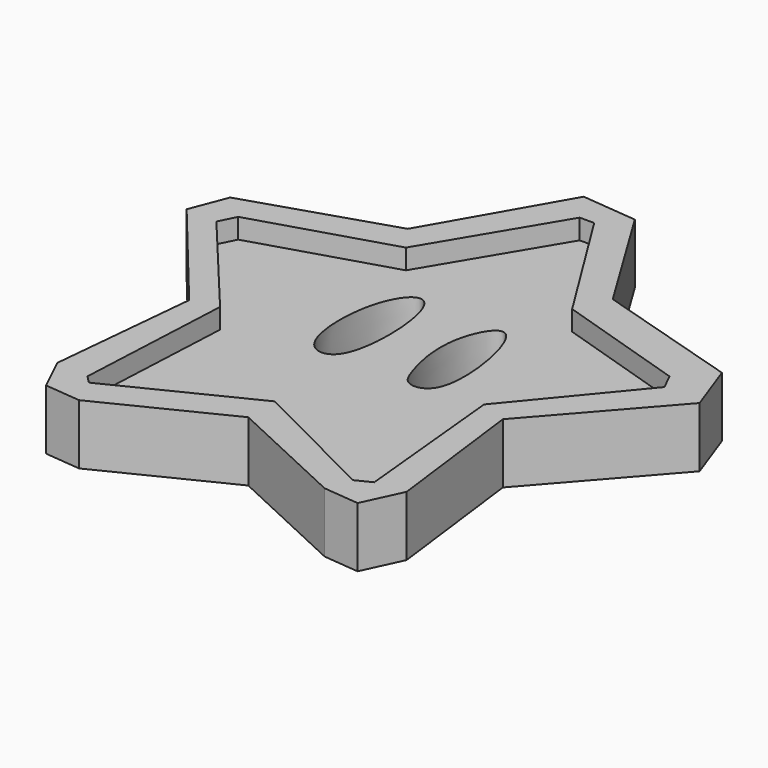
from build123d import *

# Parameters (mm, degrees)
F1_DEPTH = 4
F2_DEPTH = 6


# Not quite as in the source:
# - the program builds the solid bodies; features that only make, move or delete a surface that nothing else refers to are left out


with BuildPart() as f1:
    # F0 (on Top) → F1 (new body)
    with BuildSketch(Plane.XY):
        Polygon((21.7038933188, 40.663164109), (8.2595115528, 36.550603807), (7.4202134274, 34.8720103502), (16.652489081, 23.793278262), (15.8971212804, 8.1823393703), (16.652489081, 7.4269715697), (29.9416775716, 14.0020314224), (43.0064387619, 7.4269715697), (44.5331511124, 8.1823393703), (43.0064387619, 23.793278262), (52.1547831595, 34.8720103502), (51.3386978339, 36.5214419841), (38.3063703775, 40.663164109), (31.5554067492, 51.5035130084), (30.5740684422, 53.0792954037), (29.1223078966, 53.0792954037), align=None)
        with BuildLine():
            add(Edge.make_bspline(
                [(25.3811851144, 37.6416891813), (24.5993217345, 37.4863257412), (22.5300561127, 34.3153306276), (22.8365480412, 25.5837934463), (27.8864125101, 25.4534071145), (27.6429800893, 36.1332272512), (25.9635847642, 37.7574173449), (25.3811851144, 37.6416891813)],
                knots=[0, 0, 0, 0, 0.1813668972, 0.4393300523, 0.5815805793, 0.8649022066, 1, 1, 1, 1], degree=3))
        make_face(mode=Mode.SUBTRACT)
        with BuildLine():
            add(Edge.make_bspline(
                [(34.3616716564, 37.2220426798), (33.4467151003, 37.7104749668), (31.1715810093, 33.5652339009), (32.5688269727, 27.7274369068), (33.6539912936, 25.4758331021), (37.7493894328, 26.2185759497), (35.846752744, 36.4292601731), (34.3616716564, 37.2220426798)],
                knots=[0, 0, 0, 0, 0.1841149483, 0.4213807172, 0.554620993, 0.7011599886, 1, 1, 1, 1], degree=3))
        make_face(mode=Mode.SUBTRACT)
    extrude(amount=F1_DEPTH)

    # F0 (on Top) → F2 (join)
    with BuildSketch(Plane.XY):
        Polygon((27.1650796672, 56.0378708923), (19.8419597, 43.2266667485), (5.7267113589, 38.7097857893), (4.3151844293, 35.039819777), (14.0547072515, 23.1830105186), (12.6431845129, 8.5031520575), (14.3370144069, 4.974339623), (17.900740458, 4.6316741696), (30.0049390644, 10.6204394251), (42.1440564096, 4.974339623), (45.7077824607, 4.6316741696), (47.5078485906, 8.5031520575), (45.7077824607, 22.7595549077), (55.9770017862, 34.4752110541), (54.1420131922, 39.5567007363), (39.7444628179, 43.9324304461), (32.6868370175, 55.5069334805), align=None)
        Polygon((7.4202134274, 34.8720103502), (8.2595115528, 36.550603807), (21.7038933188, 40.663164109), (29.1223078966, 53.0792954037), (30.5740684422, 53.0792954037), (31.5554067492, 51.5035130084), (38.3063703775, 40.663164109), (51.3386978339, 36.5214419841), (52.1547831595, 34.8720103502), (43.0064387619, 23.793278262), (44.5331511124, 8.1823393703), (43.0064387619, 7.4269715697), (29.9416775716, 14.0020314224), (16.652489081, 7.4269715697), (15.8971212804, 8.1823393703), (16.652489081, 23.793278262), align=None, mode=Mode.SUBTRACT)
    extrude(amount=F2_DEPTH)


solid = f1.part
